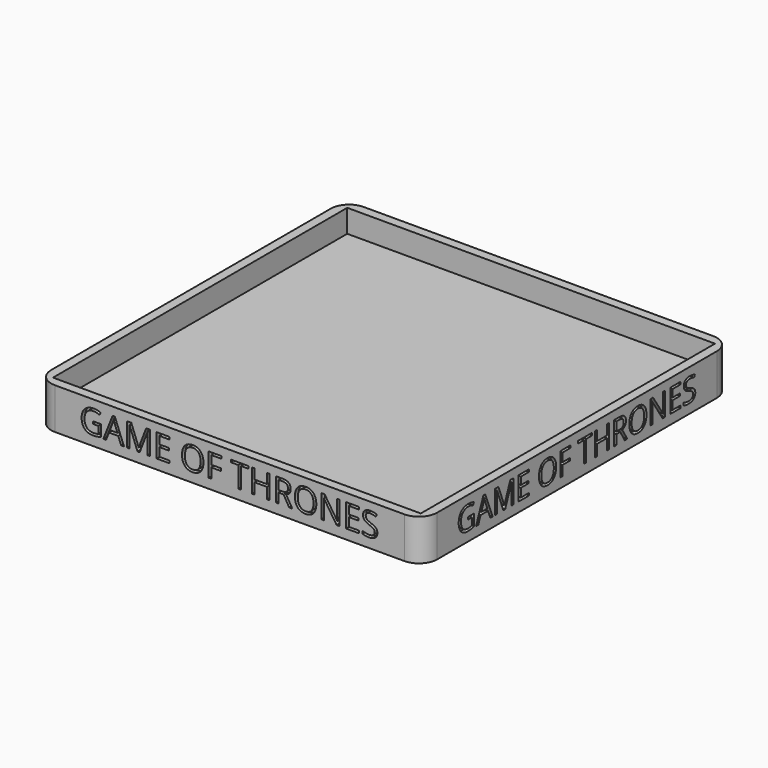
from build123d import *

# Parameters (mm, degrees)
F0_W         = 107.188
F0_H         = 107.188
F1_DEPTH     = 11.43
F2_R         = 5.08
F3_W         = 102.108
F3_H         = 102.108
F4_DEPTH     = 6.35
F5_TEXT_SIZE = 9.0506086255
F6_DEPTH     = 1.27
F9_TEXT_SIZE = 9.0506086255
F10_DEPTH    = 1.27
F8_TEXT_SIZE = 9.0506086255
F11_DEPTH    = 1.27
F7_TEXT_SIZE = 9.0506086255
F12_DEPTH    = 1.27


# Not quite as in the source:
# - Text() gives the source's letters only with a copy of the font that has no kerning and outlines rounded to 1/6400 em; it was checked with that copy


with BuildPart() as f1:
    # F0 (on Top) → F1 (new body)
    with BuildSketch(Plane.XY):
        Rectangle(F0_W, F0_H)
    extrude(amount=-F1_DEPTH)

    # F2
    f2_edges = [f1.edges().sort_by_distance(p)[0] for p in [
        (-53.594, 53.594, -5.715),
        (-53.594, -53.594, -5.715),
        (53.594, 53.594, -5.715),
        (53.594, -53.594, -5.715),
    ]]
    fillet(f2_edges, radius=F2_R)

    # F3 (on face) → F4 (cut)
    with BuildSketch(Plane.XY):
        Rectangle(F3_W, F3_H)
    extrude(amount=-F4_DEPTH, mode=Mode.SUBTRACT)

    # F5 (on face) → F6 (cut)
    with BuildSketch(Plane(origin=(-53.594, 0, 0), x_dir=(0, -1, 0), z_dir=(-1, 0, 0))):
        with Locations((-41.3141772151, -9.0289432555)):
            Text('GAME OF THRONES', F5_TEXT_SIZE, font='Open Sans', text_align=(TextAlign.LEFT, TextAlign.BOTTOM))
    extrude(amount=-F6_DEPTH, mode=Mode.SUBTRACT)

    # F9 (on face) → F10 (cut)
    with BuildSketch(Plane.XZ.offset(53.594)):
        with Locations((-41.6315793991, -8.7376013398)):
            Text('GAME OF THRONES', F9_TEXT_SIZE, font='Open Sans', text_align=(TextAlign.LEFT, TextAlign.BOTTOM))
    extrude(amount=-F10_DEPTH, mode=Mode.SUBTRACT)

    # F8 (on face) → F11 (cut)
    with BuildSketch(Plane.YZ.offset(53.594)):
        with Locations((-41.6236076531, -8.7884031236)):
            Text('GAME OF THRONES', F8_TEXT_SIZE, font='Open Sans', text_align=(TextAlign.LEFT, TextAlign.BOTTOM))
    extrude(amount=-F11_DEPTH, mode=Mode.SUBTRACT)

    # F7 (on face) → F12 (cut)
    with BuildSketch(Plane(origin=(0, 53.594, 0), x_dir=(-1, 0, 0), z_dir=(0, 1, 0))):
        with Locations((-41.5942911059, -8.7905116379)):
            Text('GAME OF THRONES', F7_TEXT_SIZE, font='Open Sans', text_align=(TextAlign.LEFT, TextAlign.BOTTOM))
    extrude(amount=-F12_DEPTH, mode=Mode.SUBTRACT)


solid = f1.part
